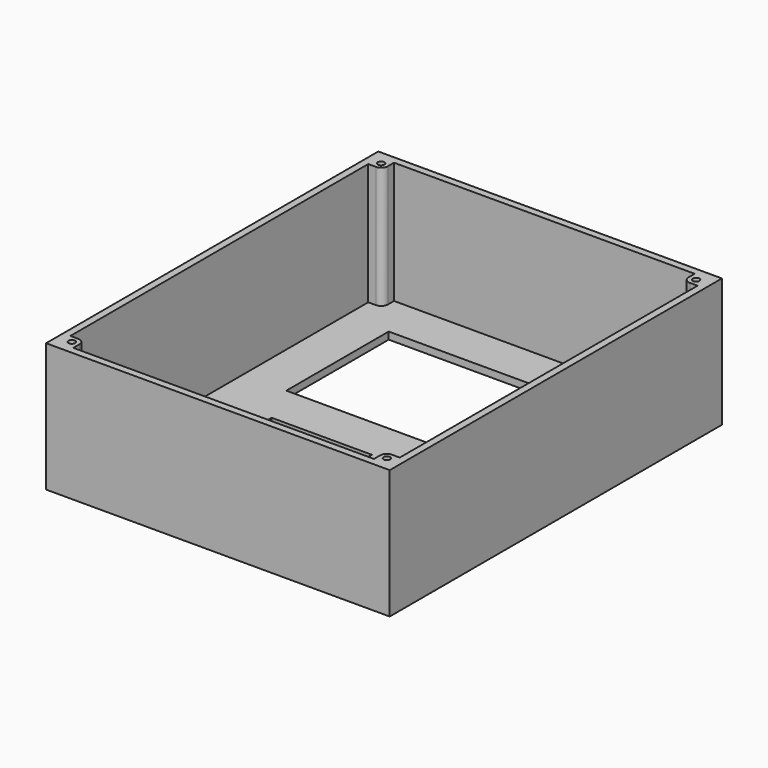
from build123d import *

# Parameters (mm, degrees)
F4_W      = 120
F4_H      = 145
F5_DEPTH  = 45
F6_T      = -2.5
F8_W      = 35
F8_H      = 45
F8_W_2    = 21.5
F8_H_2    = 29.6
F7_W      = 84.7
F7_H      = 44.7
F9_DEPTH  = 2.5
F10_W     = 5
F10_H     = 5
F11_DEPTH = 42.5
F12_R     = 1.15
F13_DEPTH = 36
F14_R     = 2.3


with BuildPart() as f5:
    # F4 (on Top) → F5 (new body)
    with BuildSketch(Plane.XY):
        Rectangle(F4_W, F4_H)
    extrude(amount=F5_DEPTH)

    # F6
    f6_openings = [f5.faces().sort_by_distance(p)[0] for p in [
        (0, 0, 45),
    ]]
    offset(amount=F6_T, openings=f6_openings)

    # F8 (on face) + F7 (on face) → F9 (cut)
    with BuildSketch(Plane.XY.offset(2.5)):
        with Locations((-18, -27.2)):
            Rectangle(F8_W, F8_H)
        with Locations((32.25, -21.4211801112)):
            Rectangle(F8_W_2, F8_H_2)
    with BuildSketch(Plane.XY.offset(2.5)):
        with Locations((0, 32.65)):
            Rectangle(F7_W, F7_H)
    extrude(amount=-F9_DEPTH, mode=Mode.SUBTRACT)

    # F10 (on face) → F11 (join)
    with BuildSketch(Plane.XY.offset(2.5)):
        with Locations((-55, 67.5)):
            Rectangle(F10_W, F10_H)
        with Locations((-55, -67.5)):
            Rectangle(F10_W, F10_H)
        with Locations((55, -67.5)):
            Rectangle(F10_W, F10_H)
        with Locations((55, 67.5)):
            Rectangle(F10_W, F10_H)
    extrude(amount=F11_DEPTH)

    # F12 (on face) → F13 (cut)
    with BuildSketch(Plane.XY.offset(45)):
        with Locations((-55, 67.5)):
            Circle(F12_R)
        with Locations((55, 67.5)):
            Circle(F12_R)
        with Locations((55, -67.5)):
            Circle(F12_R)
        with Locations((-55, -67.5)):
            Circle(F12_R)
    extrude(amount=-F13_DEPTH, mode=Mode.SUBTRACT)

    # F14
    f14_edges = [f5.edges().sort_by_distance(p)[0] for p in [
        (-52.5, 65, 23.75),
        (52.5, 65, 23.75),
        (52.5, -65, 23.75),
        (-52.5, -65, 23.75),
    ]]
    fillet(f14_edges, radius=F14_R)


solid = f5.part
